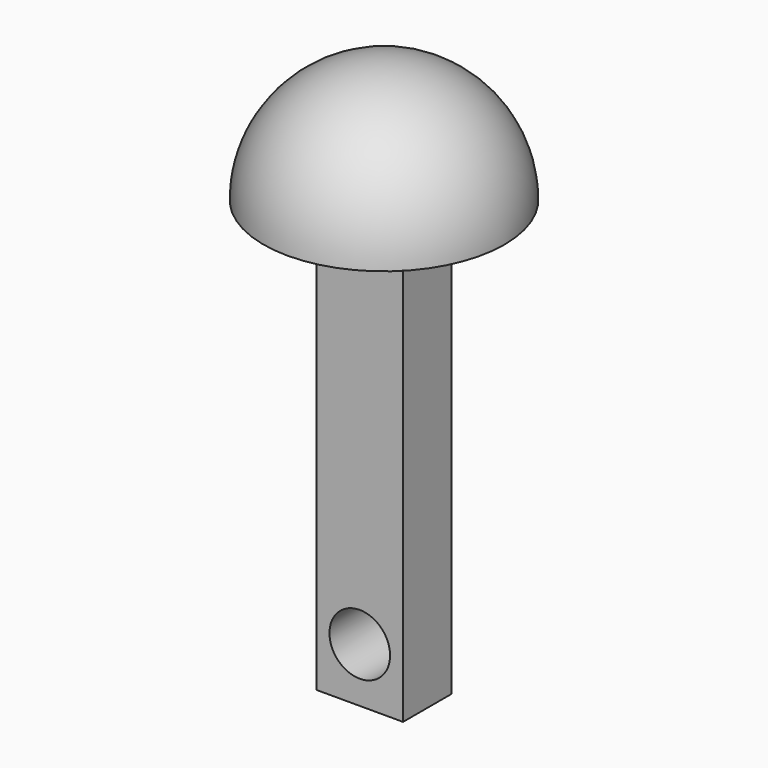
from build123d import *

# Parameters (mm, degrees)
F0_R          = 3.5
F1_DEPTH      = 3.5
F2_ANGLE_BACK = 90
F2_ANGLE      = 180


# Not quite as in the source:
# - a feature of the source that left no trace in its solid (it failed there, or was rolled back) is left out


with BuildPart() as f1:
    # F0 (on Front) → F1 (new body, symmetric)
    with BuildSketch(Plane.XZ):
        with BuildLine():
            ThreePointArc((-4.4455649331, -9.5285820105), (-9.4455649331, -10.4578883784), (-14.4455649331, -9.5285820105))
            Line((-14.4455649331, -9.5285820105), (-14.4455649331, -46.5423427522))
            Line((-14.4455649331, -46.5423427522), (-4.4455649331, -46.5423427522))
            Line((-4.4455649331, -46.5423427522), (-4.4455649331, -9.5285820105))
        make_face()
        with Locations((-9.4455649331, -40.2793101966)):
            Circle(F0_R, mode=Mode.SUBTRACT)
        with BuildLine():
            Line((-4.4455649331, 3.4576572478), (-14.4455649331, 3.4576572478))
            Line((-14.4455649331, 3.4576572478), (-14.4455649331, -9.5285820105))
            ThreePointArc((-14.4455649331, -9.5285820105), (-9.4455649331, -10.4578883784), (-4.4455649331, -9.5285820105))
            Line((-4.4455649331, -9.5285820105), (-4.4455649331, 3.4576572478))
        make_face()
    extrude(amount=F1_DEPTH, both=True)

    # F0 (on Front) → F2 (revolve)
    with BuildSketch(Plane.XZ, mode=Mode.PRIVATE) as f2_sk:
        with BuildLine():
            Line((-23.3611105593, 3.4576572478), (-14.4455649331, 3.4576572478))
            Line((-14.4455649331, 3.4576572478), (-4.4455649331, 3.4576572478))
            Line((-4.4455649331, 3.4576572478), (4.469980693, 3.4576572478))
            ThreePointArc((4.469980693, 3.4576572478), (-9.4455649331, 17.3732028739), (-23.3611105593, 3.4576572478))
        make_face()
    revolve(f2_sk.sketch.rotate(Axis((-13.6577822268, 0, 3.4576572478), (-1, 0, 0)), -F2_ANGLE_BACK), axis=Axis((-13.6577822268, 0, 3.4576572478), (-1, 0, 0)), revolution_arc=F2_ANGLE)


solid = f1.part
